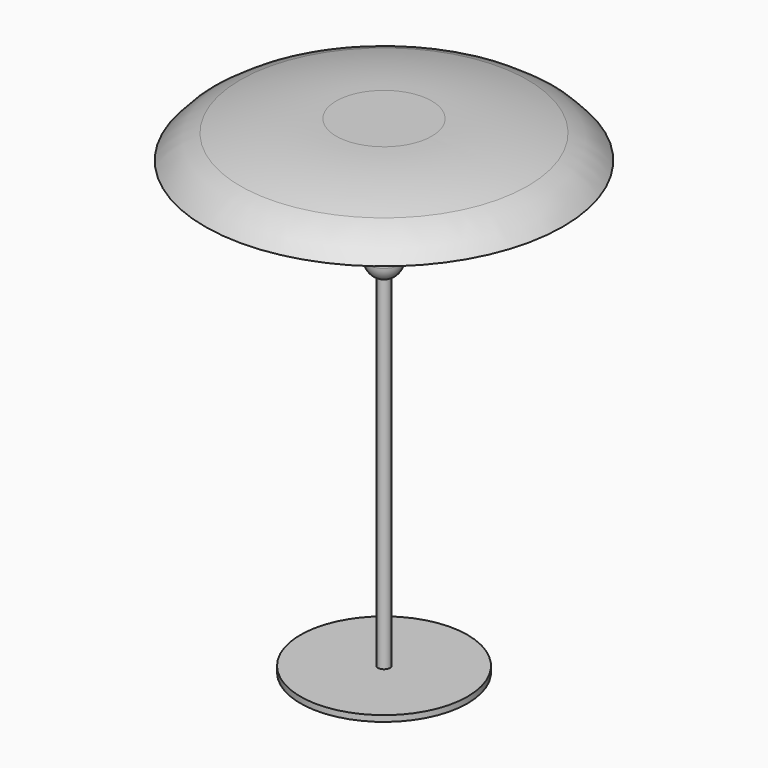
from build123d import *

# Parameters (mm, degrees)
F0_R      = 70
F1_DEPTH  = 5
F2_R      = 5
F3_DEPTH  = 5
F4_R      = 5
F5_DEPTH  = 350
F8_R      = 0.5
F9_R      = 0.49999
F11_R     = 10.5
F12_DEPTH = 27
F16_DEPTH = 5
F17_R     = 40
F17_R_2   = 18
F18_DEPTH = 2.5
F19_W     = 5
F19_H     = 10
F20_DEPTH = 70
F23_DEPTH = 2.5


# Not quite as in the source:
# - a fillet or chamfer that OpenCascade refuses, or shapes differently, is made with other operations: its cross-section is extruded or revolved along the edge and cut away or added
# - a fillet or chamfer is up to 0.001 mm smaller than in the source, because OpenCascade refuses the exact size


with BuildPart() as f1:
    # F0 (on Top) → F1 (new body)
    with BuildSketch(Plane.XY):
        Circle(F0_R)
    extrude(amount=F1_DEPTH)

    # F2 (on face) → F3 (cut, through all)
    with BuildSketch(Plane.XY.offset(5)):
        Circle(F2_R)
    extrude(amount=-F3_DEPTH, mode=Mode.SUBTRACT)


with BuildPart() as f5:
    # F4 (on Top) → F5 (new body)
    with BuildSketch(Plane.XY):
        Circle(F4_R)
    extrude(amount=F5_DEPTH)

    # F6 (on Front) → F7 (revolve)
    with BuildSketch(Plane.XZ):
        with BuildLine():
            Line((13.5, 350), (0, 350))
            Line((0, 350), (0, 291.5))
            ThreePointArc((0, 291.5), (9.545941546, 295.454058454), (13.5, 305))
            Line((13.5, 305), (13.5, 325))
            Line((13.5, 325), (18.5, 325))
            Line((18.5, 325), (18.5, 326))
            Line((18.5, 326), (13.5, 326))
            Line((13.5, 326), (13.5, 330.6318867207))
            Line((13.5, 330.6318867207), (13.5, 350))
        make_face()
    revolve(axis=Axis((0, 0, 320.75), (0, 0, -1)))

    # F8
    f8_edges = [f5.edges().sort_by_distance(p)[0] for p in [
        (-18.5, 0, 326),
    ]]
    fillet(f8_edges, radius=F8_R)

    # F9 (radius 0.5 in the source; OpenCascade refuses exactly that, so slightly less here)
    f9_edges = [f5.edges().sort_by_distance(p)[0] for p in [
        (-18.5, 0, 325),
    ]]
    fillet(f9_edges, radius=F9_R)

    # F10: chamfer of 1 x 2 on 1 edges, made by hand

    # F10_s1 → F10_t2 (revolve, cut)
    with BuildSketch(Plane.XZ):
        Polygon((13.5, 348), (12.5, 350), (13.5, 350), align=None)
    revolve(axis=Axis((0, 0, 350), (0, 0, -1)), mode=Mode.SUBTRACT)

    # F11 (on face) → F12 (cut)
    with BuildSketch(Plane.XY.offset(350)):
        Circle(F11_R)
    extrude(amount=-F12_DEPTH, mode=Mode.SUBTRACT)


with BuildPart() as f14:
    # F13 (on Front) → F14 (revolve)
    with BuildSketch(Plane.XZ):
        Polygon((13.5, 329), (18, 329), (18, 331.5), (15.5, 331.5), (15.5, 336.5), (13.5, 336.5), align=None)
    revolve(axis=Axis((0, 0, 328.6638983499), (0, 0, -1)))

    # F15 (on face) → F16 (cut)
    with BuildSketch(Plane.XY.offset(336.5)):
        with BuildLine():
            ThreePointArc((-14.1599545935, 6.3044179677), (-15.1612878114, 3.2226312077), (-15.5, 0))
            Line((-15.5, 0), (-14.5, 0))
            ThreePointArc((-14.5, 0), (-14.1831402106, 3.0147195169), (-13.2464091358, 5.8976813246))
            Line((-13.2464091358, 5.8976813246), (-14.1599545935, 6.3044179677))
        make_face()
        with BuildLine():
            ThreePointArc((-7.75, 13.4233937587), (-10.3715243986, 11.5187447949), (-12.5397634128, 9.1106714105))
            Line((-12.5397634128, 9.1106714105), (-11.7307464184, 8.5228861582))
            ThreePointArc((-11.7307464184, 8.5228861582), (-9.7023937922, 10.7755999694), (-7.25, 12.5573683549))
            Line((-7.25, 12.5573683549), (-7.75, 13.4233937587))
        make_face()
        with BuildLine():
            ThreePointArc((1.6201911806, 15.4150893782), (-1.6201911806, 15.4150893782), (-4.7897634128, 14.7413760026))
            Line((-4.7897634128, 14.7413760026), (-4.4807464184, 13.7903194863))
            ThreePointArc((-4.4807464184, 13.7903194863), (-1.5156627174, 14.4205674828), (1.5156627174, 14.4205674828))
            Line((1.5156627174, 14.4205674828), (1.6201911806, 15.4150893782))
        make_face()
        with BuildLine():
            ThreePointArc((4.4807464184, 13.7903194863), (7.25, 12.5573683549), (9.7023937922, 10.7755999694))
            Line((9.7023937922, 10.7755999694), (10.3715243986, 11.5187447949))
            ThreePointArc((10.3715243986, 11.5187447949), (7.75, 13.4233937587), (4.7897634128, 14.7413760026))
            Line((4.7897634128, 14.7413760026), (4.4807464184, 13.7903194863))
        make_face()
        with BuildLine():
            ThreePointArc((11.7307464184, 8.5228861582), (13.2464091358, 5.8976813246), (14.1831402106, 3.0147195169))
            Line((14.1831402106, 3.0147195169), (15.1612878114, 3.2226312077))
            ThreePointArc((15.1612878114, 3.2226312077), (14.1599545935, 6.3044179677), (12.5397634128, 9.1106714105))
            Line((12.5397634128, 9.1106714105), (11.7307464184, 8.5228861582))
        make_face()
        with BuildLine():
            ThreePointArc((14.5, 0), (14.1831402106, -3.0147195169), (13.2464091358, -5.8976813246))
            Line((13.2464091358, -5.8976813246), (14.1599545935, -6.3044179677))
            ThreePointArc((14.1599545935, -6.3044179677), (15.1612878114, -3.2226312077), (15.5, 0))
            Line((15.5, 0), (14.5, 0))
        make_face()
        with BuildLine():
            ThreePointArc((11.7307464184, -8.5228861582), (9.7023937922, -10.7755999694), (7.25, -12.5573683549))
            Line((7.25, -12.5573683549), (7.75, -13.4233937587))
            ThreePointArc((7.75, -13.4233937587), (10.3715243986, -11.5187447949), (12.5397634128, -9.1106714105))
            Line((12.5397634128, -9.1106714105), (11.7307464184, -8.5228861582))
        make_face()
        with BuildLine():
            ThreePointArc((4.4807464184, -13.7903194863), (1.5156627174, -14.4205674828), (-1.5156627174, -14.4205674828))
            Line((-1.5156627174, -14.4205674828), (-1.6201911806, -15.4150893782))
            ThreePointArc((-1.6201911806, -15.4150893782), (1.6201911806, -15.4150893782), (4.7897634128, -14.7413760026))
            Line((4.7897634128, -14.7413760026), (4.4807464184, -13.7903194863))
        make_face()
        with BuildLine():
            Line((-9.7023937922, -10.7755999694), (-10.3715243986, -11.5187447949))
            ThreePointArc((-10.3715243986, -11.5187447949), (-7.75, -13.4233937587), (-4.7897634128, -14.7413760026))
            Line((-4.7897634128, -14.7413760026), (-4.4807464184, -13.7903194863))
            ThreePointArc((-4.4807464184, -13.7903194863), (-7.25, -12.5573683549), (-9.7023937922, -10.7755999694))
        make_face()
        with BuildLine():
            Line((-14.1831402106, -3.0147195169), (-15.1612878114, -3.2226312077))
            ThreePointArc((-15.1612878114, -3.2226312077), (-14.1599545935, -6.3044179677), (-12.5397634128, -9.1106714105))
            Line((-12.5397634128, -9.1106714105), (-11.7307464184, -8.5228861582))
            ThreePointArc((-11.7307464184, -8.5228861582), (-13.2464091358, -5.8976813246), (-14.1831402106, -3.0147195169))
        make_face()
    extrude(amount=-F16_DEPTH, mode=Mode.SUBTRACT)


with BuildPart() as f18:
    # F17 (on face) → F18 (new body)
    with BuildSketch(Plane.XY.offset(326)):
        Circle(F17_R)
        Circle(F17_R_2, mode=Mode.SUBTRACT)
    extrude(amount=F18_DEPTH)

    # F19 (on face) → F20 (join)
    with BuildSketch(Plane.XY.offset(328.5)):
        Polygon((-23.8935008815, -22.8342823752), (-29.629265245, -14.6427619323), (-33.7250254664, -17.5106441141), (-27.9892611029, -25.702164557), align=None)
        with Locations((-35.1696164037, 0)):
            Rectangle(F19_W, F19_H)
        Polygon((-29.3397514128, 15.2145595729), (-23.4462210519, 23.2933156581), (-27.4855990945, 26.2400808386), (-33.3791294554, 18.1613247534), align=None)
        Polygon((-14.7361226495, 29.5829431467), (-5.2136437961, 32.6362031237), (-6.7402737846, 37.3974425504), (-16.2627526379, 34.3441825734), align=None)
        Polygon((5.5298433074, 32.5841168203), (15.0222697431, 29.4386692588), (16.5949935239, 34.1848824766), (7.1025670882, 37.3303300382), align=None)
        Polygon((23.6709737035, 23.0648832621), (29.4858944163, 14.9293625594), (33.5536547677, 17.8368229159), (27.7387340548, 25.9723436185), align=None)
        Polygon((32.7165612627, 4.6829963815), (32.6196000458, -5.3165335336), (37.6193650034, -5.3650141421), (37.7163262202, 4.634515773), align=None)
        Polygon((29.1908499743, -15.4983261593), (23.2192640573, -23.5195580869), (27.2298800211, -26.5053510454), (33.2014659381, -18.4841191178), align=None)
        Polygon((14.44859011, -29.7244357356), (4.8969541137, -32.6852210696), (6.3773467807, -37.4610390678), (15.928982777, -34.5002537337), align=None)
        Polygon((-5.8455229195, -32.5289670565), (-15.3070044883, -29.2916276359), (-16.9256741986, -34.0223684203), (-7.4641926298, -37.2597078408), align=None)
    extrude(amount=F20_DEPTH)

    # F23 (add): a face of the model
    f23_faces = [f5.part.faces().sort_by_distance(p)[0] for p in [
        (-17.4908831175, 0, 326),
    ]]
    extrude(f23_faces, amount=F23_DEPTH)


with BuildPart() as f22:
    # F21 (on Front) → F22 (revolve)
    with BuildSketch(Plane.XZ):
        with BuildLine():
            Line((0, 408.5), (0, 398.5))
            Line((0, 398.5), (40, 398.5))
            ThreePointArc((40, 398.5), (95.9834153044, 393.2301430306), (150, 377.6057147391))
            ThreePointArc((150, 377.6057147391), (136.9404665109, 390.2755901139), (120.4141683044, 397.8886463043))
            ThreePointArc((120.4141683044, 397.8886463043), (80.5556386072, 405.8357124988), (40, 408.5))
            Line((40, 408.5), (0, 408.5))
        make_face()
    revolve(axis=Axis((0, 0, 403.5), (0, 0, -1)))


solid = Compound([f1.part, f5.part, f14.part, f18.part, f22.part])
